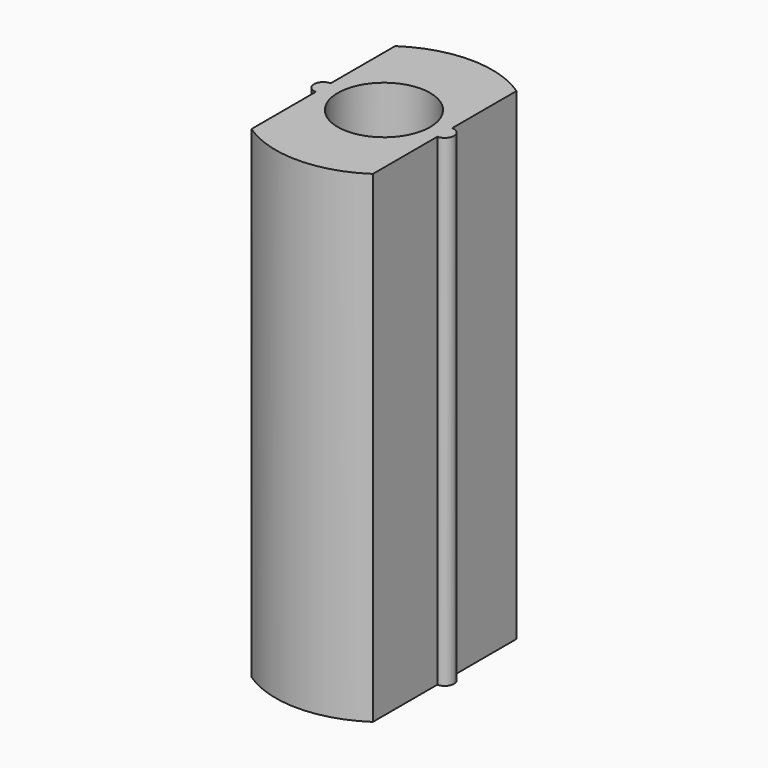
from build123d import *

# Parameters (mm, degrees)
F0_R     = 3.6
F1_DEPTH = 37.6
F2_R     = 0.725
F3_DEPTH = 37.6


# Not quite as in the source:
# - a pattern or mirror of a feature is missing from the dataset's text; its kind, count and spacing are read off the source's solid


with BuildPart() as f1:
    # F0 (on Top) → F1 (new body)
    with BuildSketch(Plane.XY):
        with BuildLine():
            Line((4.7331279298, -7), (4.7331279298, 7))
            ThreePointArc((4.7331279298, 7), (0, 8.45), (-4.7331279298, 7))
            Line((-4.7331279298, 7), (-4.7331279298, -7))
            ThreePointArc((-4.7331279298, -7), (0, -8.45), (4.7331279298, -7))
        make_face()
        Circle(F0_R, mode=Mode.SUBTRACT)
    extrude(amount=F1_DEPTH)

    # F2 (on face) → F3 (join)
    with BuildSketch(Plane.XY.offset(37.6)):
        with Locations((4.7331279298, 0)):
            Circle(F2_R)
    f3 = extrude(amount=-F3_DEPTH)

    # F3_copies: F3 across plane
    add(f3.mirror(Plane(origin=(0, 0, 0), x_dir=(0, 0, -1), z_dir=(-1, 0, 0))))


solid = f1.part
